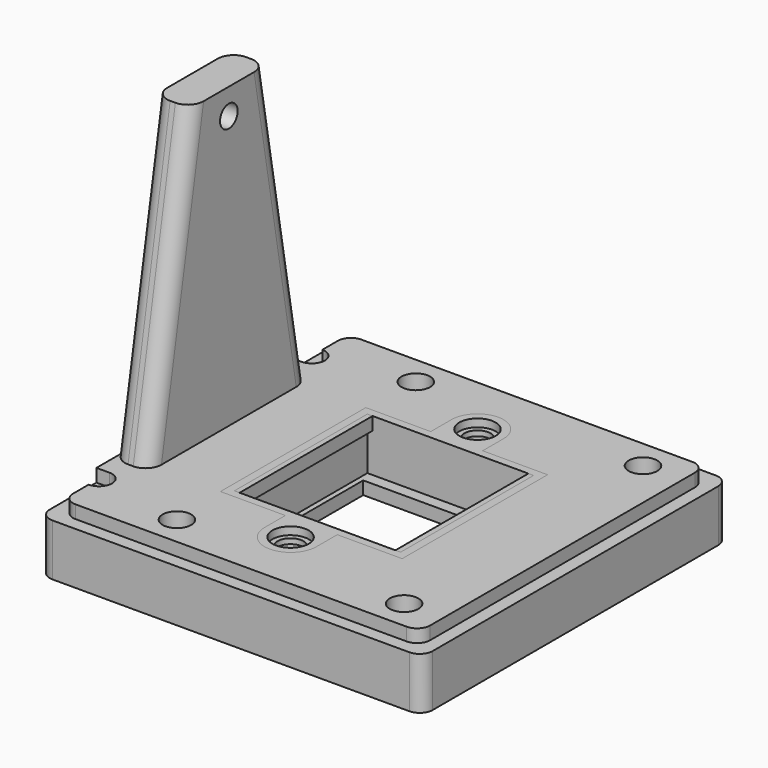
from build123d import *

# Parameters (mm, degrees)
F0_W            = 29.5
F0_H            = 29.5
F0_W_2          = 19.5
F0_H_2          = 19.5
F1_DEPTH        = 4
F2_W            = 2.8
F2_H            = 17.3
F3_DEPTH        = 24
F4_T4_DEPTH     = 150.1704583371
F4_T9_DEPTH     = 150.1704583371
F5_R            = 1.2
F2_W_2          = 12
F2_H_2          = 14
F6_DEPTH        = 1
F8_D            = 2.2
F8_DEPTH        = 20
F8_TIP          = 0.6609466809
F9_W            = 12
F9_H            = 11
F10_DEPTH       = 1
F11_R           = 1.4
F11_W           = 12.8
F11_H           = 12.8
F12_DEPTH       = 5
F14_D           = 1.7
F14_DEPTH       = 5
F14_CSINK_D     = 3.5
F14_CSINK_ANGLE = 90
F14_TIP         = 0.5107315262
F15_D           = 2.7
F15_DEPTH       = 4.2
F15_TIP         = 0.8111618357
F17_D           = 2
F17_DEPTH       = 4.2
F17_CBORE_D     = 3
F17_CBORE_DEPTH = 0.6
F17_TIP         = 0.600860619
F18_D           = 2
F18_DEPTH       = 20
F18_CBORE_D     = 3
F18_CBORE_DEPTH = 0.6
F18_TIP         = 0.600860619
F19_DEPTH       = 25
F20_R           = 1


# Not quite as in the source:
# - a fillet or chamfer that OpenCascade refuses, or shapes differently, is made with other operations: its cross-section is extruded or revolved along the edge and cut away or added
# - a pattern or mirror of a feature is missing from the dataset's text; its kind, count and spacing are read off the source's solid
# - a feature names something its author has since deleted; it is built from what else it names


with BuildPart() as f1:
    # F0 (on Top) → F1 (new body)
    with BuildSketch(Plane.XY):
        Rectangle(F0_W, F0_H)
        Rectangle(F0_W_2, F0_H_2, mode=Mode.SUBTRACT)
    extrude(amount=F1_DEPTH)

    # F2 (on face) → F3 (join)
    with BuildSketch(Plane.XY.offset(4)):
        with Locations((-13.35, 0)):
            Rectangle(F2_W, F2_H)
    extrude(amount=F3_DEPTH)

    # F4: chamfer of 5 x 28.3564090981 on 2 edges, made by hand


with BuildPart() as f4_tool2:
    # F4_s3 → F4_t4 (new body)
    with BuildSketch(Plane.YZ.offset(-88.4352291686)):
        Polygon((-8.65, -0.3564090981), (-3.65, 28), (-8.65, 28), align=None)
    extrude(amount=F4_T4_DEPTH)

    split(bisect_by=Plane.XY.offset(4), keep=Keep.TOP)


with BuildPart() as f1_1:
    add(f1.part)

    # F4_t1: cut F4_tool2
    add(f4_tool2.part, mode=Mode.SUBTRACT)


with BuildPart() as f4_tool7:
    # F4_s8 → F4_t9 (new body)
    with BuildSketch(Plane.YZ.offset(61.7352291686)):
        Polygon((8.65, -0.3564090981), (3.65, 28), (8.65, 28), align=None)
    extrude(amount=-F4_T9_DEPTH)

    split(bisect_by=Plane.XY.offset(4), keep=Keep.TOP)


with BuildPart() as f1_2:
    add(f1_1.part)

    # F4_t6: cut F4_tool7
    add(f4_tool7.part, mode=Mode.SUBTRACT)

    # F5
    f5_edges = [f1_2.edges().sort_by_distance(p)[0] for p in [
        (-11.95, -5.765924, 16),
        (-14.75, -5.765924, 16),
        (-11.95, 5.765924, 16),
        (-14.75, 5.765924, 16),
    ]]
    fillet(f5_edges, radius=F5_R)

    # F2 (on face) → F6 (join)
    with BuildSketch(Plane.XY.offset(4)):
        with BuildLine():
            Line((13.75, -13.75), (13.75, 13.75))
            Line((13.75, 13.75), (-13.75, 13.75))
            Line((-13.75, 13.75), (-13.75, 11.25))
            ThreePointArc((-13.75, 11.25), (-12.75, 10.25), (-13.75, 9.25))
            Line((-13.75, 9.25), (-14.75, 9.25))
            Line((-14.75, 9.25), (-14.75, 8.65))
            Line((-14.75, 8.65), (-11.95, 8.65))
            Line((-11.95, 8.65), (-11.95, -8.65))
            Line((-11.95, -8.65), (-14.75, -8.65))
            Line((-14.75, -8.65), (-14.75, -9.25))
            Line((-14.75, -9.25), (-13.75, -9.25))
            ThreePointArc((-13.75, -9.25), (-12.75, -10.25), (-13.75, -11.25))
            Line((-13.75, -11.25), (-13.75, -13.75))
            Line((-13.75, -13.75), (13.75, -13.75))
        make_face()
        with BuildLine():
            ThreePointArc((-2.25, 9.75), (0, 12), (2.25, 9.75))
            Line((2.25, 9.75), (9.75, 9.75))
            Line((9.75, 9.75), (9.75, -9.75))
            Line((9.75, -9.75), (2.25, -9.75))
            ThreePointArc((2.25, -9.75), (0, -12), (-2.25, -9.75))
            Line((-2.25, -9.75), (-9.75, -9.75))
            Line((-9.75, -9.75), (-9.75, 9.75))
            Line((-9.75, 9.75), (-2.25, 9.75))
        make_face(mode=Mode.SUBTRACT)
        with Locations((-13.35, 0)):
            Rectangle(F2_W, F2_H)
        with BuildLine():
            Line((9.75, 9.75), (2.25, 9.75))
            ThreePointArc((2.25, 9.75), (0, 7.5), (-2.25, 9.75))
            Line((-2.25, 9.75), (-9.75, 9.75))
            Line((-9.75, 9.75), (-9.75, -9.75))
            Line((-9.75, -9.75), (-2.25, -9.75))
            ThreePointArc((-2.25, -9.75), (0, -7.5), (2.25, -9.75))
            Line((2.25, -9.75), (9.75, -9.75))
            Line((9.75, -9.75), (9.75, 9.75))
        make_face()
        Rectangle(F2_W_2, F2_H_2, mode=Mode.SUBTRACT)
        with BuildLine():
            Line((-2.25, 9.75), (2.25, 9.75))
            ThreePointArc((2.25, 9.75), (0, 12), (-2.25, 9.75))
        make_face()
        with BuildLine():
            ThreePointArc((-2.25, 9.75), (0, 7.5), (2.25, 9.75))
            Line((2.25, 9.75), (-2.25, 9.75))
        make_face()
        with BuildLine():
            Line((-2.25, -9.75), (2.25, -9.75))
            ThreePointArc((2.25, -9.75), (0, -7.5), (-2.25, -9.75))
        make_face()
        with BuildLine():
            ThreePointArc((-2.25, -9.75), (0, -12), (2.25, -9.75))
            Line((2.25, -9.75), (-2.25, -9.75))
        make_face()
    extrude(amount=F6_DEPTH)

    # F8
    with Locations(Plane.XY.offset(5)):
        with Locations((10.75, 11.5), (10.75, -11.5), (-6.75, 11.5), (-6.75, -11.5)):
            Hole(F8_D / 2, depth=F8_DEPTH)
            with Locations((0, 0, -(F8_DEPTH + F8_TIP / 2))):  # 118° drill point
                Cone(0, F8_D / 2, F8_TIP, mode=Mode.SUBTRACT)

    # F14
    with Locations(Plane(origin=(-14.75, 0, 0), x_dir=(0, -1, 0), z_dir=(-1, 0, 0))):
        with Locations((0, 26)):
            CounterSinkHole(F14_D / 2, F14_CSINK_D / 2, depth=F14_DEPTH, counter_sink_angle=F14_CSINK_ANGLE)
            with Locations((0, 0, -(F14_DEPTH + F14_TIP / 2))):  # 118° drill point
                Cone(0, F14_D / 2, F14_TIP, mode=Mode.SUBTRACT)

    # F15
    with Locations(Plane(origin=(-14.75, 0, 0), x_dir=(0, -1, 0), z_dir=(-1, 0, 0))):
        with Locations((-12.25, 2), (12.25, 2)):
            Hole(F15_D / 2, depth=F15_DEPTH)
            with Locations((0, 0, -(F15_DEPTH + F15_TIP / 2))):  # 118° drill point
                Cone(0, F15_D / 2, F15_TIP, mode=Mode.SUBTRACT)

    # F18
    with Locations(Plane.XY.offset(5)):
        with Locations((0, 9), (0, -9)):
            CounterBoreHole(F18_D / 2, F18_CBORE_D / 2, F18_CBORE_DEPTH, depth=F18_DEPTH)
            with Locations((0, 0, -(F18_DEPTH + F18_TIP / 2))):  # 118° drill point
                Cone(0, F18_D / 2, F18_TIP, mode=Mode.SUBTRACT)

    # F2 (on face) → F19 (cut)
    with BuildSketch(Plane.XY.offset(4)):
        with BuildLine():
            ThreePointArc((-2.25, 9.75), (0, 7.5), (2.25, 9.75))
            Line((2.25, 9.75), (-2.25, 9.75))
        make_face()
        with BuildLine():
            Line((-2.25, -9.75), (2.25, -9.75))
            ThreePointArc((2.25, -9.75), (0, -7.5), (-2.25, -9.75))
        make_face()
        with BuildLine():
            ThreePointArc((-2.25, -9.75), (0, -12), (2.25, -9.75))
            Line((2.25, -9.75), (-2.25, -9.75))
        make_face()
    f19 = extrude(amount=-F19_DEPTH, mode=Mode.SUBTRACT)

    # F19_copies: F19 across plane
    add(f19.mirror(Plane.ZX), mode=Mode.SUBTRACT)

    # F20
    f20_edges = [f1_2.edges().sort_by_distance(p)[0] for p in [
        (-14.75, -14.75, 2),
        (-13.75, -13.75, 4.5),
        (13.75, -13.75, 4.5),
        (14.75, -14.75, 2),
        (13.75, 13.75, 4.5),
        (14.75, 14.75, 2),
        (-13.75, 13.75, 4.5),
        (-14.75, 14.75, 2),
    ]]
    fillet(f20_edges, radius=F20_R)


with BuildPart() as f10:
    # F9 (on Top) → F10 (new body)
    with BuildSketch(Plane.XY):
        with BuildLine():
            ThreePointArc((9.9875, -0.4998437256), (9.9968745116, -0.25), (10, 0))
            ThreePointArc((10, 0), (9.9968745116, 0.25), (9.9875, 0.4998437256))
            ThreePointArc((9.9875, 0.4998437256), (9.5, 0), (9.9875, -0.4998437256))
        make_face()
        with BuildLine():
            ThreePointArc((9.9875, 0.4998437256), (9.9968745116, 0.25), (10, 0))
            ThreePointArc((10, 0), (9.9968745116, -0.25), (9.9875, -0.4998437256))
            ThreePointArc((9.9875, -0.4998437256), (10.3491060011, -0.3579455266), (10.5, 0))
            ThreePointArc((10.5, 0), (10.3491060011, 0.3579455266), (9.9875, 0.4998437256))
        make_face()
        with BuildLine():
            ThreePointArc((9.9875, -0.4998437256), (9.5, 0), (9.9875, 0.4998437256))
            ThreePointArc((9.9875, 0.4998437256), (8.6602540378, 5), (5.4266273643, 8.3995068575))
            ThreePointArc((5.4266273643, 8.3995068575), (4.75, 8.227241336), (4.5608726357, 8.8993505831))
            ThreePointArc((4.5608726357, 8.8993505831), (3.3062354904, 9.437627185), (1.9899748742, 9.8))
            ThreePointArc((1.9899748742, 9.8), (0, 8), (-1.9899748742, 9.8))
            ThreePointArc((-1.9899748742, 9.8), (-3.3062354904, 9.437627185), (-4.5608726357, 8.8993505831))
            ThreePointArc((-4.5608726357, 8.8993505831), (-4.5154570803, 8.7836159401), (-4.5, 8.6602540378))
            ThreePointArc((-4.5, 8.6602540378), (-4.8645630814, 8.178946609), (-5.4266273643, 8.3995068575))
            ThreePointArc((-5.4266273643, 8.3995068575), (-8.6602540378, 5), (-9.9875, 0.4998437256))
            ThreePointArc((-9.9875, 0.4998437256), (-9.6420544734, 0.3491060011), (-9.5, 0))
            ThreePointArc((-9.5, 0), (-9.6420544734, -0.3491060011), (-9.9875, -0.4998437256))
            ThreePointArc((-9.9875, -0.4998437256), (-8.6602540378, -5), (-5.4266273643, -8.3995068575))
            ThreePointArc((-5.4266273643, -8.3995068575), (-4.8645630814, -8.178946609), (-4.5, -8.6602540378))
            ThreePointArc((-4.5, -8.6602540378), (-4.5154570803, -8.7836159401), (-4.5608726357, -8.8993505831))
            ThreePointArc((-4.5608726357, -8.8993505831), (-3.3062354904, -9.437627185), (-1.9899748742, -9.8))
            ThreePointArc((-1.9899748742, -9.8), (0, -8), (1.9899748742, -9.8))
            ThreePointArc((1.9899748742, -9.8), (3.3062354904, -9.437627185), (4.5608726357, -8.8993505831))
            ThreePointArc((4.5608726357, -8.8993505831), (4.75, -8.227241336), (5.4266273643, -8.3995068575))
            ThreePointArc((5.4266273643, -8.3995068575), (8.6602540378, -5), (9.9875, -0.4998437256))
        make_face()
        Rectangle(F9_W, F9_H, mode=Mode.SUBTRACT)
        with BuildLine():
            ThreePointArc((4.5608726357, 8.8993505831), (4.75, 8.227241336), (5.4266273643, 8.3995068575))
            ThreePointArc((5.4266273643, 8.3995068575), (5, 8.6602540378), (4.5608726357, 8.8993505831))
        make_face()
        with BuildLine():
            ThreePointArc((4.5608726357, 8.8993505831), (5, 8.6602540378), (5.4266273643, 8.3995068575))
            ThreePointArc((5.4266273643, 8.3995068575), (5.4813074289, 8.5248171192), (5.5, 8.6602540378))
            ThreePointArc((5.5, 8.6602540378), (5.1233619023, 9.1447969576), (4.5608726357, 8.8993505831))
        make_face()
        with BuildLine():
            ThreePointArc((5.5, -8.6602540378), (5.4813074289, -8.5248171192), (5.4266273643, -8.3995068575))
            ThreePointArc((5.4266273643, -8.3995068575), (5, -8.6602540378), (4.5608726357, -8.8993505831))
            ThreePointArc((4.5608726357, -8.8993505831), (5.1233619023, -9.1447969576), (5.5, -8.6602540378))
        make_face()
        with BuildLine():
            ThreePointArc((4.5608726357, -8.8993505831), (5, -8.6602540378), (5.4266273643, -8.3995068575))
            ThreePointArc((5.4266273643, -8.3995068575), (4.75, -8.227241336), (4.5608726357, -8.8993505831))
        make_face()
        with BuildLine():
            ThreePointArc((-1.9899748742, 9.8), (0, 8), (1.9899748742, 9.8))
            ThreePointArc((1.9899748742, 9.8), (0, 10), (-1.9899748742, 9.8))
        make_face()
        with BuildLine():
            ThreePointArc((-1.9899748742, 9.8), (0, 10), (1.9899748742, 9.8))
            ThreePointArc((1.9899748742, 9.8), (1.9974921462, 9.8998744499), (2, 10))
            ThreePointArc((2, 10), (-0.1001255501, 11.9974921462), (-1.9899748742, 9.8))
        make_face()
        with BuildLine():
            ThreePointArc((2, -10), (1.9974921462, -9.8998744499), (1.9899748742, -9.8))
            ThreePointArc((1.9899748742, -9.8), (0, -10), (-1.9899748742, -9.8))
            ThreePointArc((-1.9899748742, -9.8), (-0.1001255501, -11.9974921462), (2, -10))
        make_face()
        with BuildLine():
            ThreePointArc((-1.9899748742, -9.8), (0, -10), (1.9899748742, -9.8))
            ThreePointArc((1.9899748742, -9.8), (0, -8), (-1.9899748742, -9.8))
        make_face()
        with BuildLine():
            ThreePointArc((-4.5, 8.6602540378), (-4.5154570803, 8.7836159401), (-4.5608726357, 8.8993505831))
            ThreePointArc((-4.5608726357, 8.8993505831), (-5, 8.6602540378), (-5.4266273643, 8.3995068575))
            ThreePointArc((-5.4266273643, 8.3995068575), (-4.8645630814, 8.178946609), (-4.5, 8.6602540378))
        make_face()
        with BuildLine():
            ThreePointArc((-5.4266273643, 8.3995068575), (-5, 8.6602540378), (-4.5608726357, 8.8993505831))
            ThreePointArc((-4.5608726357, 8.8993505831), (-5.25, 9.0932667397), (-5.4266273643, 8.3995068575))
        make_face()
        with BuildLine():
            ThreePointArc((-5.4266273643, -8.3995068575), (-5.25, -9.0932667397), (-4.5608726357, -8.8993505831))
            ThreePointArc((-4.5608726357, -8.8993505831), (-5, -8.6602540378), (-5.4266273643, -8.3995068575))
        make_face()
        with BuildLine():
            ThreePointArc((-5.4266273643, -8.3995068575), (-5, -8.6602540378), (-4.5608726357, -8.8993505831))
            ThreePointArc((-4.5608726357, -8.8993505831), (-4.5154570803, -8.7836159401), (-4.5, -8.6602540378))
            ThreePointArc((-4.5, -8.6602540378), (-4.8645630814, -8.178946609), (-5.4266273643, -8.3995068575))
        make_face()
        with BuildLine():
            ThreePointArc((-9.5, 0), (-9.6420544734, 0.3491060011), (-9.9875, 0.4998437256))
            ThreePointArc((-9.9875, 0.4998437256), (-10, 0), (-9.9875, -0.4998437256))
            ThreePointArc((-9.9875, -0.4998437256), (-9.6420544734, -0.3491060011), (-9.5, 0))
        make_face()
        with BuildLine():
            ThreePointArc((-9.9875, -0.4998437256), (-10, 0), (-9.9875, 0.4998437256))
            ThreePointArc((-9.9875, 0.4998437256), (-10.5, 0), (-9.9875, -0.4998437256))
        make_face()
    extrude(amount=F10_DEPTH)

    # F17
    with Locations(Plane.XY.offset(1)):
        with Locations((0, 9), (0, -9)):
            CounterBoreHole(F17_D / 2, F17_CBORE_D / 2, F17_CBORE_DEPTH, depth=F17_DEPTH)
            with Locations((0, 0, -(F17_DEPTH + F17_TIP / 2))):  # 118° drill point
                Cone(0, F17_D / 2, F17_TIP, mode=Mode.SUBTRACT)


with BuildPart() as f12:
    # F11 (on Top) → F12 (new body)
    with BuildSketch(Plane.XY):
        with BuildLine():
            Line((-2, 7), (0, 7))
            ThreePointArc((0, 7), (-1.4142135624, 7.5857864376), (-2, 9))
            Line((-2, 9), (-2, 7))
        make_face()
        with BuildLine():
            ThreePointArc((-2, 9), (-1.4142135624, 7.5857864376), (0, 7))
            ThreePointArc((0, 7), (1.4142135624, 7.5857864376), (2, 9))
            ThreePointArc((2, 9), (0, 11), (-2, 9))
        make_face()
        with Locations((0, 9)):
            Circle(F11_R, mode=Mode.SUBTRACT)
        with BuildLine():
            Line((0, 7), (2, 7))
            Line((2, 7), (2, 9))
            ThreePointArc((2, 9), (1.4142135624, 7.5857864376), (0, 7))
        make_face()
        Polygon((2, -7), (7, -7), (7, 7), (2, 7), (0, 7), (-2, 7), (-7, 7), (-7, -7), (-2, -7), (0, -7), align=None)
        Rectangle(F11_W, F11_H, mode=Mode.SUBTRACT)
        with BuildLine():
            Line((2, -9), (2, -7))
            Line((2, -7), (0, -7))
            ThreePointArc((0, -7), (1.4142135624, -7.5857864376), (2, -9))
        make_face()
        with BuildLine():
            ThreePointArc((2, -9), (1.4142135624, -7.5857864376), (0, -7))
            ThreePointArc((0, -7), (-1.4142135624, -7.5857864376), (-2, -9))
            ThreePointArc((-2, -9), (0, -11), (2, -9))
        make_face()
        with Locations((0, -9)):
            Circle(F11_R, mode=Mode.SUBTRACT)
        with BuildLine():
            ThreePointArc((-2, -9), (-1.4142135624, -7.5857864376), (0, -7))
            Line((0, -7), (-2, -7))
            Line((-2, -7), (-2, -9))
        make_face()
    extrude(amount=F12_DEPTH)


solid = Compound([f1_2.part, f10.part, f12.part])
